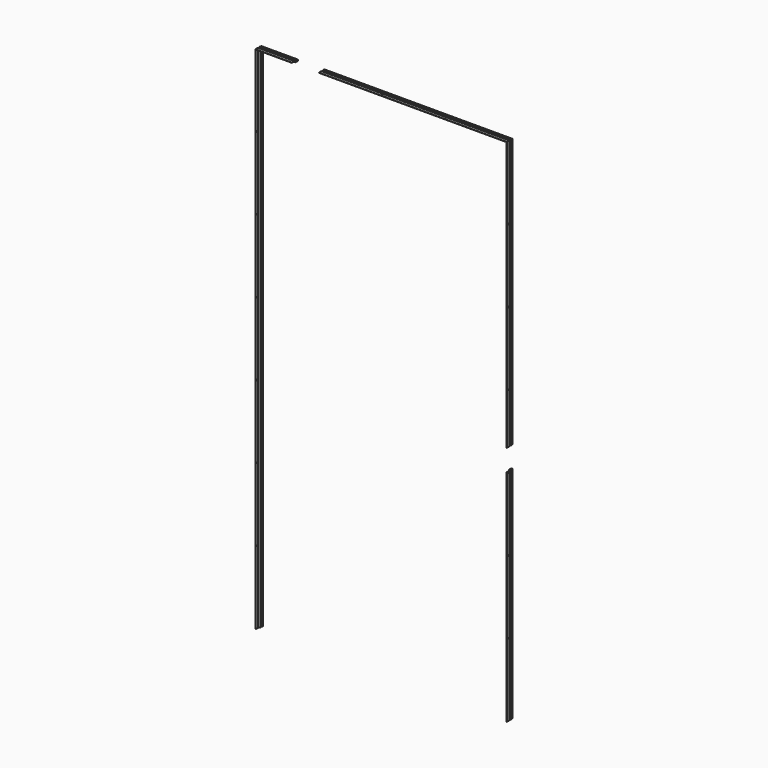
from build123d import *

# Parameters (mm, degrees)
F1_R           = 2.2225
F2_DEPTH       = 2114.55
F3_DEPTH       = 2114.55
F8_DEPTH       = 31.751
F8_DEPTH_BACK  = 3537
F11_COUNT      = 2
F11_ANGLE      = 270
F13_DEPTH      = 4440
F13_DEPTH_BACK = 31.751
F14_W          = 145.8515469776
F14_H          = 88.9
F15_DEPTH      = 60.96
F16_R          = 1.5875
F17_DEPTH      = 1041.401
F17_DEPTH_BACK = 3733
F18_R          = 1.5875
F19_DEPTH      = 3733
F19_DEPTH_BACK = 2114.551
F20_W          = 111.6735892
F20_H          = 130.9275875603
F21_DEPTH      = 31.751
F21_DEPTH_BACK = 3733


# Not quite as in the source:
# - an extrude ends at something that could not be found from the text; its depth is read off the source's solid


with BuildPart() as f2:
    # F1 (on Top) → F2 (new body)
    with BuildSketch(Plane.XY):
        with BuildLine():
            Line((-3.175, 21.4488888889), (-3.175, 23.4244444444))
            Line((-3.175, 23.4244444444), (-2.1166666667, 23.4244444444))
            Line((-2.1166666667, 23.4244444444), (-2.1166666667, 25.825369343))
            ThreePointArc((-2.1166666667, 25.825369343), (-3.7041666667, 31.75), (-5.2916666667, 25.825369343))
            Line((-5.2916666667, 25.825369343), (-5.2916666667, 23.4244444444))
            Line((-5.2916666667, 23.4244444444), (-4.2333333333, 23.4244444444))
            Line((-4.2333333333, 23.4244444444), (-4.2333333333, 21.4488888889))
            Line((-4.2333333333, 21.4488888889), (-5.2916666667, 21.4488888889))
            Line((-5.2916666667, 21.4488888889), (-5.2916666667, 19.4733333333))
            Line((-5.2916666667, 19.4733333333), (-2.1166666667, 19.4733333333))
            Line((-2.1166666667, 19.4733333333), (-2.1166666667, 21.4488888889))
            Line((-2.1166666667, 21.4488888889), (-3.175, 21.4488888889))
        make_face()
        with Locations((-3.7041666667, 28.575)):
            Circle(F1_R, mode=Mode.SUBTRACT)
    extrude(amount=F2_DEPTH)


with BuildPart() as f3:
    # F0 (on Top) → F3 (new body)
    with BuildSketch(Plane.XY):
        Polygon((-1.0583333333, 0), (0, 0), (0, 12.7), (-5.2916666667, 18.415), (0, 18.415), (0, 26.19375), (-1.0583333333, 26.19375), (-1.0583333333, 24.13), (-2.1166666667, 25.4), (-2.1166666667, 23.4244444444), (-3.175, 23.4244444444), (-3.175, 21.4488888889), (-2.1166666667, 21.4488888889), (-2.1166666667, 19.4733333333), (-5.2916666667, 19.4733333333), (-5.2916666667, 21.4488888889), (-4.2333333333, 21.4488888889), (-4.2333333333, 23.4244444444), (-5.2916666667, 23.4244444444), (-5.2916666667, 25.4), (-6.35, 24.13), (-6.35, 18.0002713829), (-1.0583333333, 12.2852713829), align=None)
    extrude(amount=F3_DEPTH)


with BuildPart() as f6_1:
    # F6: instance of F2
    add(f2.part.mirror(Plane.YZ.offset(-520.7)))


with BuildPart() as f6_2:
    # F6: instance of F3
    add(f3.part.mirror(Plane.YZ.offset(-520.7)))


with BuildPart() as f8_tool:
    # F7 (on Front) → F8 (new body, two sides)
    with BuildSketch(Plane.XZ) as f8_sk:
        Polygon((0, 2114.55), (-1041.4, 2114.55), (-520.7, 1593.85), align=None)
    extrude(amount=-F8_DEPTH)
    extrude(f8_sk.sketch, amount=F8_DEPTH_BACK)


with BuildPart() as f2_1:
    add(f2.part)

    # F8: cut by f8_tool
    add(f8_tool.part, mode=Mode.SUBTRACT)


with BuildPart() as f3_1:
    add(f3.part)

    # F8: cut by f8_tool
    add(f8_tool.part, mode=Mode.SUBTRACT)


with BuildPart() as f6_1_1:
    add(f6_1.part)

    # F8: cut by f8_tool
    add(f8_tool.part, mode=Mode.SUBTRACT)


with BuildPart() as f6_2_1:
    add(f6_2.part)

    # F8: cut by f8_tool
    add(f8_tool.part, mode=Mode.SUBTRACT)


with BuildPart() as f11_1:
    # F11: instance of F2
    add(f2_1.part.rotate(Axis((-520.7, 198.7161487341, 1593.85), (0, 1, 0)), 1 * F11_ANGLE / (F11_COUNT - 1)))


with BuildPart() as f11_2:
    # F11: instance of F3
    add(f3_1.part.rotate(Axis((-520.7, 198.7161487341, 1593.85), (0, 1, 0)), 1 * F11_ANGLE / (F11_COUNT - 1)))


with BuildPart() as f13_tool:
    # F12 (on Front) → F13 (new body, two sides)
    with BuildSketch(Plane.XZ) as f13_sk:
        Polygon((0, 2114.55), (-520.7, 1593.85), (1152.4028778076, 1593.85), (1152.4028778076, 3266.9528778076), align=None)
    extrude(amount=F13_DEPTH)
    extrude(f13_sk.sketch, amount=-F13_DEPTH_BACK)


with BuildPart() as f11_1_1:
    add(f11_1.part)

    # F13: cut by f13_tool
    add(f13_tool.part, mode=Mode.SUBTRACT)


with BuildPart() as f11_2_1:
    add(f11_2.part)

    # F13: cut by f13_tool
    add(f13_tool.part, mode=Mode.SUBTRACT)

    # F18 (on Top) → F19 (cut, two sides)
    with BuildSketch(Plane.XY) as f19_sk:
        with Locations((-781.05, 6.35)):
            Circle(F18_R)
        with Locations((-520.7, 6.35)):
            Circle(F18_R)
        with Locations((-260.35, 6.35)):
            Circle(F18_R)
    extrude(amount=-F19_DEPTH, mode=Mode.SUBTRACT)
    extrude(f19_sk.sketch, amount=F19_DEPTH_BACK, mode=Mode.SUBTRACT)


with BuildPart() as f15_tool:
    # F14 (on Front) → F15 (new body)
    with BuildSketch(Plane.XZ):
        with Locations((13.1394341588, 954.826005)):
            Rectangle(F14_W, F14_H)
    extrude(amount=-F15_DEPTH)


with BuildPart() as f2_2:
    add(f2_1.part)

    # F15: cut by f15_tool
    add(f15_tool.part, mode=Mode.SUBTRACT)


with BuildPart() as f3_2:
    add(f3_1.part)

    # F15: cut by f15_tool
    add(f15_tool.part, mode=Mode.SUBTRACT)


with BuildPart() as f17_tool:
    # F16 (on Right) → F17 (new body, two sides)
    with BuildSketch(Plane.YZ) as f17_sk:
        with Locations((6.35, 1812.4714285714)):
            Circle(F16_R)
        with Locations((6.35, 1510.3928571429)):
            Circle(F16_R)
        with Locations((6.35, 1208.3142857143)):
            Circle(F16_R)
        with Locations((6.35, 906.2357142857)):
            Circle(F16_R)
        with Locations((6.35, 604.1571428571)):
            Circle(F16_R)
        with Locations((6.35, 302.0785714286)):
            Circle(F16_R)
    extrude(amount=-F17_DEPTH)
    extrude(f17_sk.sketch, amount=F17_DEPTH_BACK)


with BuildPart() as f3_3:
    add(f3_2.part)

    # F17: cut by f17_tool
    add(f17_tool.part, mode=Mode.SUBTRACT)


with BuildPart() as f6_2_2:
    add(f6_2_1.part)

    # F17: cut by f17_tool
    add(f17_tool.part, mode=Mode.SUBTRACT)


with BuildPart() as f21_tool:
    # F20 (on Front) → F21 (new body, two sides)
    with BuildSketch(Plane.XZ) as f21_sk:
        with Locations((-834.8777054, 2140.0084495544)):
            Rectangle(F20_W, F20_H)
    extrude(amount=-F21_DEPTH)
    extrude(f21_sk.sketch, amount=F21_DEPTH_BACK)


with BuildPart() as f11_1_2:
    add(f11_1_1.part)

    # F21: cut by f21_tool
    add(f21_tool.part, mode=Mode.SUBTRACT)


with BuildPart() as f11_2_2:
    add(f11_2_1.part)

    # F21: cut by f21_tool
    add(f21_tool.part, mode=Mode.SUBTRACT)


solid = Compound([f6_1_1.part, f2_2.part, f3_3.part, f6_2_2.part, f11_1_2.part, f11_2_2.part])
